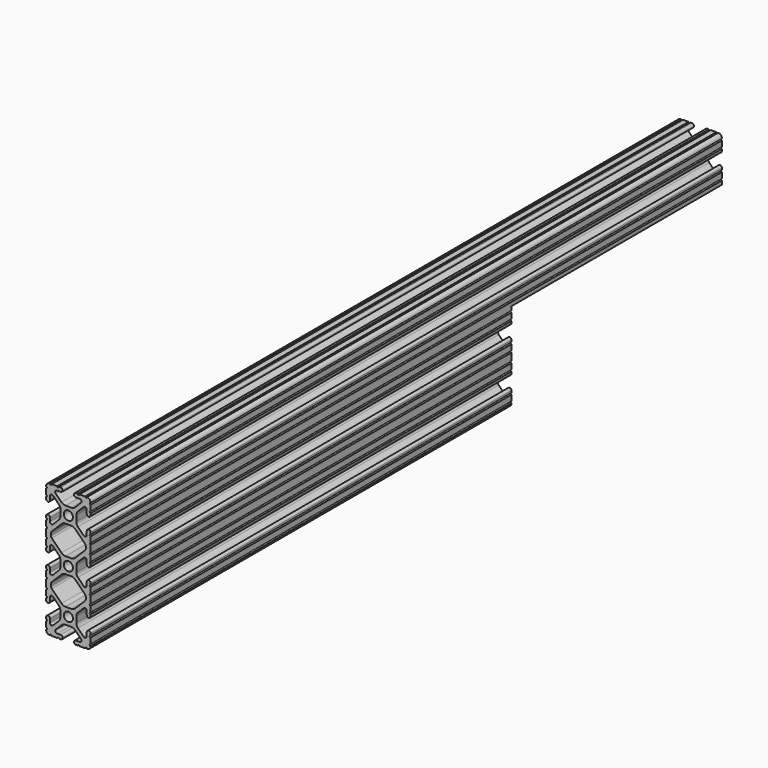
from build123d import *

# Parameters (mm, degrees)
F1_DEPTH = 450
F2_W     = 53.2047543675
F2_H     = 56.1891395271
F3_DEPTH = 150


# Not quite as in the source:
# - ends of sketch curves that miss each other by under 0.0002 mm in the source are joined


with BuildPart() as f1:
    # F0 (on Front) → F1 (new body)
    with BuildSketch(Plane.XZ):
        with BuildLine():
            ThreePointArc((-9.5504, 38.1), (-10.0584, 37.592), (-10.5664, 38.1))
            ThreePointArc((-10.5664, 38.1), (-12.0826749161, 37.4826749161), (-12.699997541, 35.9664000298))
            ThreePointArc((-12.699997541, 35.9664000298), (-12.192, 35.4584), (-12.7, 34.9504))
            Line((-12.7, 34.9504), (-12.7, 31.7246))
            ThreePointArc((-12.7, 31.7246), (-12.192, 31.2166), (-12.7, 30.7086))
            Line((-12.7, 30.7086), (-12.7, 29.7023028))
            ThreePointArc((-12.7, 29.7023028), (-11.5951, 28.5974028), (-10.4902, 29.7023028))
            Line((-10.4902, 29.7023028), (-10.4902, 31.8747902))
            ThreePointArc((-10.4902, 31.8747902), (-9.8630063673, 32.813451805), (-8.7557795103, 32.5932106897))
            Line((-8.7557795103, 32.5932106897), (-5.4384448, 29.2758622))
            ThreePointArc((-5.4384448, 29.2758622), (-4.7501824843, 28.2458268978), (-4.5085, 27.030807))
            Line((-4.5085, 27.030807), (-4.5085, 23.769193))
            ThreePointArc((-4.5085, 23.769193), (-4.7501824843, 22.5541731022), (-5.4384359697, 21.5241289697))
            Line((-5.4384359697, 21.5241289697), (-8.7557864, 18.2067962))
            ThreePointArc((-8.7557864, 18.2067962), (-9.8630063673, 17.986548195), (-10.4902, 18.9252098))
            Line((-10.4902, 18.9252098), (-10.4902, 21.0976972))
            ThreePointArc((-10.4902, 21.0976972), (-11.5951, 22.2025972), (-12.7, 21.0976972))
            Line((-12.7, 21.0976972), (-12.7, 20.0914))
            ThreePointArc((-12.7, 20.0914), (-12.192, 19.5834), (-12.7, 19.0754))
            Line((-12.7, 19.0754), (-12.7, 15.8496))
            ThreePointArc((-12.7, 15.8496), (-12.192, 15.3416), (-12.7, 14.8336))
            Line((-12.7, 14.8336), (-12.7, 10.5664))
            ThreePointArc((-12.7, 10.5664), (-12.192, 10.0584), (-12.7, 9.5504))
            Line((-12.7, 9.5504), (-12.7, 6.3246))
            ThreePointArc((-12.7, 6.3246), (-12.192, 5.8166), (-12.7, 5.3086))
            Line((-12.7, 5.3086), (-12.7, 4.3023028))
            ThreePointArc((-12.7, 4.3023028), (-11.5951, 3.1974028), (-10.4902, 4.3023028))
            Line((-10.4902, 4.3023028), (-10.4902, 6.4747902))
            ThreePointArc((-10.4902, 6.4747902), (-9.8630063673, 7.413451805), (-8.7557795103, 7.1932106897))
            Line((-8.7557795103, 7.1932106897), (-5.4384448, 3.8758622))
            ThreePointArc((-5.4384448, 3.8758622), (-4.7501824843, 2.8458268978), (-4.5085, 1.630807))
            Line((-4.5085, 1.630807), (-4.5085, -1.630807))
            ThreePointArc((-4.5085, -1.630807), (-4.7501824843, -2.8458268978), (-5.4384359697, -3.8758710303))
            Line((-5.4384359697, -3.8758710303), (-8.7557864, -7.1932038))
            ThreePointArc((-8.7557864, -7.1932038), (-9.8630063673, -7.413451805), (-10.4902, -6.4747902))
            Line((-10.4902, -6.4747902), (-10.4902, -4.3023028))
            ThreePointArc((-10.4902, -4.3023028), (-11.5951, -3.1974028), (-12.7, -4.3023028))
            Line((-12.7, -4.3023028), (-12.7, -5.3086))
            ThreePointArc((-12.7, -5.3086), (-12.192, -5.8166), (-12.7, -6.3246))
            Line((-12.7, -6.3246), (-12.7, -9.5504))
            ThreePointArc((-12.7, -9.5504), (-12.192, -10.0584), (-12.7, -10.5664))
            Line((-12.7, -10.5664), (-12.7, -14.8336))
            ThreePointArc((-12.7, -14.8336), (-12.192, -15.3416), (-12.7, -15.8496))
            Line((-12.7, -15.8496), (-12.7, -19.0754))
            ThreePointArc((-12.7, -19.0754), (-12.192, -19.5834), (-12.7, -20.0914))
            Line((-12.7, -20.0914), (-12.7, -21.0976972))
            ThreePointArc((-12.7, -21.0976972), (-11.5951, -22.2025972), (-10.4902, -21.0976972))
            Line((-10.4902, -21.0976972), (-10.4902, -18.9252098))
            ThreePointArc((-10.4902, -18.9252098), (-9.8630063673, -17.986548195), (-8.7557795103, -18.2067893103))
            Line((-8.7557795103, -18.2067893103), (-5.4384448, -21.5241378))
            ThreePointArc((-5.4384448, -21.5241378), (-4.7501824843, -22.5541731022), (-4.5085, -23.769193))
            Line((-4.5085, -23.769193), (-4.5085, -27.030807))
            ThreePointArc((-4.5085, -27.030807), (-4.7501824843, -28.2458268978), (-5.4384359697, -29.2758710303))
            Line((-5.4384359697, -29.2758710303), (-8.7557864, -32.5932038))
            ThreePointArc((-8.7557864, -32.5932038), (-9.8630063673, -32.813451805), (-10.4902, -31.8747902))
            Line((-10.4902, -31.8747902), (-10.4902, -29.7023028))
            ThreePointArc((-10.4902, -29.7023028), (-11.5951, -28.5974028), (-12.7, -29.7023028))
            Line((-12.7, -29.7023028), (-12.7, -30.7086))
            ThreePointArc((-12.7, -30.7086), (-12.192, -31.2166), (-12.7, -31.7246))
            Line((-12.7, -31.7246), (-12.7, -34.9504))
            ThreePointArc((-12.7, -34.9504), (-12.192, -35.4584), (-12.7, -35.9664))
            ThreePointArc((-12.7, -35.9664), (-12.0826749161, -37.4826749161), (-10.5664000298, -38.099997541))
            ThreePointArc((-10.5664000298, -38.099997541), (-10.0584, -37.592), (-9.5504, -38.1))
            Line((-9.5504, -38.1), (-6.3246, -38.1))
            ThreePointArc((-6.3246, -38.1), (-5.8166, -37.592), (-5.3086, -38.1))
            Line((-5.3086, -38.1), (-4.3023028, -38.1))
            ThreePointArc((-4.3023028, -38.1), (-3.1974028, -36.9951), (-4.3023028, -35.8902))
            Line((-4.3023028, -35.8902), (-6.4747902, -35.8902))
            ThreePointArc((-6.4747902, -35.8902), (-7.413451805, -35.2630063673), (-7.1932106897, -34.1557795103))
            Line((-7.1932106897, -34.1557795103), (-3.8758622, -30.8384448))
            ThreePointArc((-3.8758622, -30.8384448), (-2.8458268978, -30.1501824843), (-1.630807, -29.9085))
            Line((-1.630807, -29.9085), (1.630807, -29.9085))
            ThreePointArc((1.630807, -29.9085), (2.8458268978, -30.1501824843), (3.8758710303, -30.8384359697))
            Line((3.8758710303, -30.8384359697), (7.1932038, -34.1557864))
            ThreePointArc((7.1932038, -34.1557864), (7.413451805, -35.2630063673), (6.4747902, -35.8902))
            Line((6.4747902, -35.8902), (4.3023028, -35.8902))
            ThreePointArc((4.3023028, -35.8902), (3.1974028, -36.9951), (4.3023028, -38.1))
            Line((4.3023028, -38.1), (5.3086, -38.1))
            ThreePointArc((5.3086, -38.1), (5.8166, -37.592), (6.3246, -38.1))
            Line((6.3246, -38.1), (9.5504, -38.1))
            ThreePointArc((9.5504, -38.1), (10.0584, -37.592), (10.5664, -38.1))
            ThreePointArc((10.5664, -38.1), (12.0826749161, -37.4826749161), (12.699997541, -35.9664000298))
            ThreePointArc((12.699997541, -35.9664000298), (12.192, -35.4584), (12.7, -34.9504))
            Line((12.7, -34.9504), (12.7, -31.7246))
            ThreePointArc((12.7, -31.7246), (12.192, -31.2166), (12.7, -30.7086))
            Line((12.7, -30.7086), (12.7, -29.7023028))
            ThreePointArc((12.7, -29.7023028), (11.5951, -28.5974028), (10.4902, -29.7023028))
            Line((10.4902, -29.7023028), (10.4902, -31.8747902))
            ThreePointArc((10.4902, -31.8747902), (9.8630063673, -32.813451805), (8.7557795103, -32.5932106897))
            Line((8.7557795103, -32.5932106897), (5.4384448, -29.2758622))
            ThreePointArc((5.4384448, -29.2758622), (4.7501824843, -28.2458268978), (4.5085, -27.030807))
            Line((4.5085, -27.030807), (4.5085, -23.769193))
            ThreePointArc((4.5085, -23.769193), (4.7501824843, -22.5541731022), (5.4384359697, -21.5241289697))
            Line((5.4384359697, -21.5241289697), (8.7557864, -18.2067962))
            ThreePointArc((8.7557864, -18.2067962), (9.8630063673, -17.986548195), (10.4902, -18.9252098))
            Line((10.4902, -18.9252098), (10.4902, -21.0976972))
            ThreePointArc((10.4902, -21.0976972), (11.5951, -22.2025972), (12.7, -21.0976972))
            Line((12.7, -21.0976972), (12.7, -20.0914))
            ThreePointArc((12.7, -20.0914), (12.192, -19.5834), (12.7, -19.0754))
            Line((12.7, -19.0754), (12.7, -15.8496))
            ThreePointArc((12.7, -15.8496), (12.192, -15.3416), (12.7, -14.8336))
            Line((12.7, -14.8336), (12.7, -10.5664))
            ThreePointArc((12.7, -10.5664), (12.192, -10.0584), (12.7, -9.5504))
            Line((12.7, -9.5504), (12.7, -6.3246))
            ThreePointArc((12.7, -6.3246), (12.192, -5.8166), (12.7, -5.3086))
            Line((12.7, -5.3086), (12.7, -4.3023028))
            ThreePointArc((12.7, -4.3023028), (11.5951, -3.1974028), (10.4902, -4.3023028))
            Line((10.4902, -4.3023028), (10.4902, -6.4747902))
            ThreePointArc((10.4902, -6.4747902), (9.8630063673, -7.413451805), (8.7557795103, -7.1932106897))
            Line((8.7557795103, -7.1932106897), (5.4384448, -3.8758622))
            ThreePointArc((5.4384448, -3.8758622), (4.7501824843, -2.8458268978), (4.5085, -1.630807))
            Line((4.5085, -1.630807), (4.5085, 1.630807))
            ThreePointArc((4.5085, 1.630807), (4.7501824843, 2.8458268978), (5.4384359697, 3.8758710303))
            Line((5.4384359697, 3.8758710303), (8.7557864, 7.1932038))
            ThreePointArc((8.7557864, 7.1932038), (9.8630063673, 7.413451805), (10.4902, 6.4747902))
            Line((10.4902, 6.4747902), (10.4902, 4.3023028))
            ThreePointArc((10.4902, 4.3023028), (11.5951, 3.1974028), (12.7, 4.3023028))
            Line((12.7, 4.3023028), (12.7, 5.3086))
            ThreePointArc((12.7, 5.3086), (12.192, 5.8166), (12.7, 6.3246))
            Line((12.7, 6.3246), (12.7, 9.5504))
            ThreePointArc((12.7, 9.5504), (12.192, 10.0584), (12.7, 10.5664))
            Line((12.7, 10.5664), (12.7, 14.8336))
            ThreePointArc((12.7, 14.8336), (12.192, 15.3416), (12.7, 15.8496))
            Line((12.7, 15.8496), (12.7, 19.0754))
            ThreePointArc((12.7, 19.0754), (12.192, 19.5834), (12.7, 20.0914))
            Line((12.7, 20.0914), (12.7, 21.0976972))
            ThreePointArc((12.7, 21.0976972), (11.5951, 22.2025972), (10.4902, 21.0976972))
            Line((10.4902, 21.0976972), (10.4902, 18.9252098))
            ThreePointArc((10.4902, 18.9252098), (9.8630063673, 17.986548195), (8.7557795103, 18.2067893103))
            Line((8.7557795103, 18.2067893103), (5.4384448, 21.5241378))
            ThreePointArc((5.4384448, 21.5241378), (4.7501824843, 22.5541731022), (4.5085, 23.769193))
            Line((4.5085, 23.769193), (4.5085, 27.030807))
            ThreePointArc((4.5085, 27.030807), (4.7501824843, 28.2458268978), (5.4384359697, 29.2758710303))
            Line((5.4384359697, 29.2758710303), (8.7557864, 32.5932038))
            ThreePointArc((8.7557864, 32.5932038), (9.8630063673, 32.813451805), (10.4902, 31.8747902))
            Line((10.4902, 31.8747902), (10.4902, 29.7023028))
            ThreePointArc((10.4902, 29.7023028), (11.5951, 28.5974028), (12.7, 29.7023028))
            Line((12.7, 29.7023028), (12.7, 30.7086))
            ThreePointArc((12.7, 30.7086), (12.192, 31.2166), (12.7, 31.7246))
            Line((12.7, 31.7246), (12.7, 34.9504))
            ThreePointArc((12.7, 34.9504), (12.192, 35.4584), (12.7, 35.9664))
            ThreePointArc((12.7, 35.9664), (12.0826749161, 37.4826749161), (10.5664000298, 38.099997541))
            ThreePointArc((10.5664000298, 38.099997541), (10.0584, 37.592), (9.5504, 38.1))
            Line((9.5504, 38.1), (6.3246, 38.1))
            ThreePointArc((6.3246, 38.1), (5.8166, 37.592), (5.3086, 38.1))
            Line((5.3086, 38.1), (4.3023028, 38.1))
            ThreePointArc((4.3023028, 38.1), (3.1974028, 36.9951), (4.3023028, 35.8902))
            Line((4.3023028, 35.8902), (6.4747902, 35.8902))
            ThreePointArc((6.4747902, 35.8902), (7.413451805, 35.2630063673), (7.1932106897, 34.1557795103))
            Line((7.1932106897, 34.1557795103), (3.8758622, 30.8384448))
            ThreePointArc((3.8758622, 30.8384448), (2.8458268978, 30.1501824843), (1.630807, 29.9085))
            Line((1.630807, 29.9085), (-1.630807, 29.9085))
            ThreePointArc((-1.630807, 29.9085), (-2.8458268978, 30.1501824843), (-3.8758710303, 30.8384359697))
            Line((-3.8758710303, 30.8384359697), (-7.1932038, 34.1557864))
            ThreePointArc((-7.1932038, 34.1557864), (-7.413451805, 35.2630063673), (-6.4747902, 35.8902))
            Line((-6.4747902, 35.8902), (-4.3023028, 35.8902))
            ThreePointArc((-4.3023028, 35.8902), (-3.1974028, 36.9951), (-4.3023028, 38.1))
            Line((-4.3023028, 38.1), (-5.3086, 38.1))
            ThreePointArc((-5.3086, 38.1), (-5.8166, 37.592), (-6.3246, 38.1))
            Line((-6.3246, 38.1), (-9.5504, 38.1))
        make_face()
        with BuildLine():
            ThreePointArc((-2.6035, -25.4), (0, -22.7965), (2.6035, -25.4))
            ThreePointArc((2.6035, -25.4), (0, -28.0035), (-2.6035, -25.4))
        make_face(mode=Mode.SUBTRACT)
        with BuildLine():
            Line((-9.4701614, -11.0327186), (-3.8758622, -5.4384448))
            ThreePointArc((-3.8758622, -5.4384448), (-2.8458268978, -4.7501824843), (-1.630807, -4.5085))
            Line((-1.630807, -4.5085), (1.630807, -4.5085))
            ThreePointArc((1.630807, -4.5085), (2.8458268978, -4.7501824843), (3.8758710303, -5.4384359697))
            Line((3.8758710303, -5.4384359697), (9.4701614, -11.0327186))
            ThreePointArc((9.4701614, -11.0327186), (9.8115254878, -11.5436301307), (9.9314, -12.14628))
            Line((9.9314, -12.14628), (9.9314, -13.25372))
            ThreePointArc((9.9314, -13.25372), (9.8115254878, -13.8563698693), (9.470151759, -14.367271759))
            Line((9.470151759, -14.367271759), (3.8758622, -19.9615552))
            ThreePointArc((3.8758622, -19.9615552), (2.8458268978, -20.6498175157), (1.630807, -20.8915))
            Line((1.630807, -20.8915), (-1.630807, -20.8915))
            ThreePointArc((-1.630807, -20.8915), (-2.8458268978, -20.6498175157), (-3.8758710303, -19.9615640303))
            Line((-3.8758710303, -19.9615640303), (-9.4701614, -14.3672814))
            ThreePointArc((-9.4701614, -14.3672814), (-9.8115254878, -13.8563698693), (-9.9314, -13.25372))
            Line((-9.9314, -13.25372), (-9.9314, -12.14628))
            ThreePointArc((-9.9314, -12.14628), (-9.8115254878, -11.5436301307), (-9.4701614, -11.0327186))
        make_face(mode=Mode.SUBTRACT)
        with BuildLine():
            ThreePointArc((-2.6035, 0), (0, 2.6035), (2.6035, 0))
            ThreePointArc((2.6035, 0), (0, -2.6035), (-2.6035, 0))
        make_face(mode=Mode.SUBTRACT)
        with BuildLine():
            Line((-9.4701614, 14.3672814), (-3.8758622, 19.9615552))
            ThreePointArc((-3.8758622, 19.9615552), (-2.8458268978, 20.6498175157), (-1.630807, 20.8915))
            Line((-1.630807, 20.8915), (1.630807, 20.8915))
            ThreePointArc((1.630807, 20.8915), (2.8458268978, 20.6498175157), (3.8758710303, 19.9615640303))
            Line((3.8758710303, 19.9615640303), (9.4701614, 14.3672814))
            ThreePointArc((9.4701614, 14.3672814), (9.8115254878, 13.8563698693), (9.9314, 13.25372))
            Line((9.9314, 13.25372), (9.9314, 12.14628))
            ThreePointArc((9.9314, 12.14628), (9.8115254878, 11.5436301307), (9.470151759, 11.032728241))
            Line((9.470151759, 11.032728241), (3.8758622, 5.4384448))
            ThreePointArc((3.8758622, 5.4384448), (2.8458268978, 4.7501824843), (1.630807, 4.5085))
            Line((1.630807, 4.5085), (-1.630807, 4.5085))
            ThreePointArc((-1.630807, 4.5085), (-2.8458268978, 4.7501824843), (-3.8758710303, 5.4384359697))
            Line((-3.8758710303, 5.4384359697), (-9.4701614, 11.0327186))
            ThreePointArc((-9.4701614, 11.0327186), (-9.8115254878, 11.5436301307), (-9.9314, 12.14628))
            Line((-9.9314, 12.14628), (-9.9314, 13.25372))
            ThreePointArc((-9.9314, 13.25372), (-9.8115254878, 13.8563698693), (-9.4701614, 14.3672814))
        make_face(mode=Mode.SUBTRACT)
        with BuildLine():
            ThreePointArc((-2.6035, 25.4), (0, 28.0035), (2.6035, 25.4))
            ThreePointArc((2.6035, 25.4), (0, 22.7965), (-2.6035, 25.4))
        make_face(mode=Mode.SUBTRACT)
    extrude(amount=F1_DEPTH)

    # F2 (on face) → F3 (cut)
    with BuildSketch(Plane(origin=(0, 0, 0), x_dir=(-1, 0, 0), z_dir=(0, 1, 0))):
        with Locations((-2.4376483634, -15.3945697635)):
            Rectangle(F2_W, F2_H)
    extrude(amount=-F3_DEPTH, mode=Mode.SUBTRACT)


solid = f1.part
